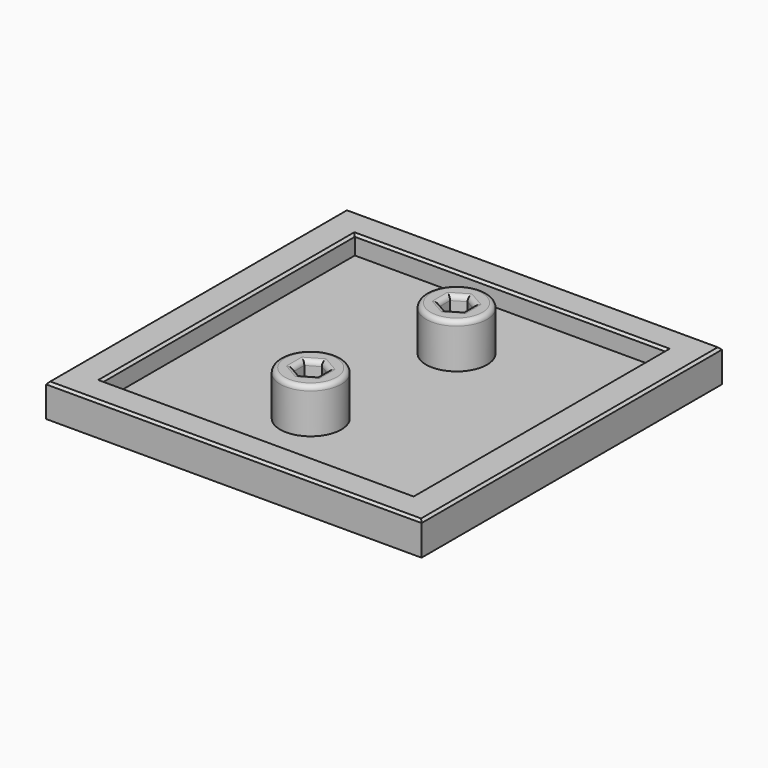
from build123d import *

# Parameters (mm, degrees)
F0_W     = 80
F0_H     = 80
F0_R     = 6.5
F1_DEPTH = 3
F2_DEPTH = 12.5
F3_R     = 1
F4_W     = 80
F4_H     = 80
F4_W_2   = 66.2
F4_H_2   = 67.2
F5_DEPTH = 4
F6_SIZE  = 0.5


# Not quite as in the source:
# - a feature names something its author has since deleted; it is built from what else it names


with BuildPart() as f1:
    # F0 (on Top) → F1 (new body)
    with BuildSketch(Plane.XY):
        Rectangle(F0_W, F0_H)
        with Locations((-2.17, -16.8)):
            Circle(F0_R, mode=Mode.SUBTRACT)
        with Locations((2.17, 16.617)):
            Circle(F0_R, mode=Mode.SUBTRACT)
        with Locations((2.17, 16.617)):
            Circle(F0_R)
        Polygon((-0.3917684664, 18.0686688068), (2.1462978314, 19.5613909739), (4.7080662978, 18.1097221671), (4.7317684664, 15.1653311932), (2.1937021686, 13.6726090261), (-0.3680662978, 15.1242778329), align=None, mode=Mode.SUBTRACT)
        Polygon((4.7080662978, 18.1097221671), (2.1462978314, 19.5613909739), (-0.3917684664, 18.0686688068), (-0.3680662978, 15.1242778329), (2.1937021686, 13.6726090261), (4.7317684664, 15.1653311932), align=None)
        with Locations((-2.17, -16.8)):
            Circle(F0_R)
        Polygon((-2.17, -13.8555136271), (0.38, -15.3277568136), (0.38, -18.2722431864), (-2.17, -19.7444863729), (-4.72, -18.2722431864), (-4.72, -15.3277568136), align=None, mode=Mode.SUBTRACT)
        Polygon((0.38, -18.2722431864), (0.38, -15.3277568136), (-2.17, -13.8555136271), (-4.72, -15.3277568136), (-4.72, -18.2722431864), (-2.17, -19.7444863729), align=None)
    extrude(amount=F1_DEPTH)

    # F0 (on Top) → F2 (join)
    with BuildSketch(Plane.XY):
        with Locations((2.17, 16.617)):
            Circle(F0_R)
        Polygon((-0.3917684664, 18.0686688068), (2.1462978314, 19.5613909739), (4.7080662978, 18.1097221671), (4.7317684664, 15.1653311932), (2.1937021686, 13.6726090261), (-0.3680662978, 15.1242778329), align=None, mode=Mode.SUBTRACT)
        with Locations((-2.17, -16.8)):
            Circle(F0_R)
        Polygon((-2.17, -13.8555136271), (0.38, -15.3277568136), (0.38, -18.2722431864), (-2.17, -19.7444863729), (-4.72, -18.2722431864), (-4.72, -15.3277568136), align=None, mode=Mode.SUBTRACT)
    extrude(amount=F2_DEPTH)

    # F3
    f3_edges = [f1.edges().sort_by_distance(p)[0] for p in [
        (-4.33, 16.617, 12.5),
        (0.877265, 18.81503, 12.5),
        (3.427182, 18.835557, 12.5),
        (4.719917, 16.637527, 12.5),
        (3.462735, 14.41897, 12.5),
        (0.912818, 14.398443, 12.5),
        (-0.379917, 16.596473, 12.5),
        (-8.67, -16.8, 12.5),
        (-0.895, -14.591635, 12.5),
        (0.38, -16.8, 12.5),
        (-0.895, -19.008365, 12.5),
        (-3.445, -19.008365, 12.5),
        (-4.72, -16.8, 12.5),
        (-3.445, -14.591635, 12.5),
    ]]
    fillet(f3_edges, radius=F3_R)

    # F4 (on face) → F5 (join)
    with BuildSketch(Plane.XY.offset(3)):
        Rectangle(F4_W, F4_H)
        Rectangle(F4_W_2, F4_H_2, mode=Mode.SUBTRACT)
    extrude(amount=F5_DEPTH)

    # F6
    f6_edges = [f1.edges().sort_by_distance(p)[0] for p in [
        (0, -40, 7),
        (40, 0, 7),
        (0, 40, 7),
        (-40, 0, 7),
        (0, 33.6, 7),
        (33.1, 0, 7),
        (0, -33.6, 7),
        (-33.1, 0, 7),
    ]]
    chamfer(f6_edges, length=F6_SIZE)


solid = f1.part
